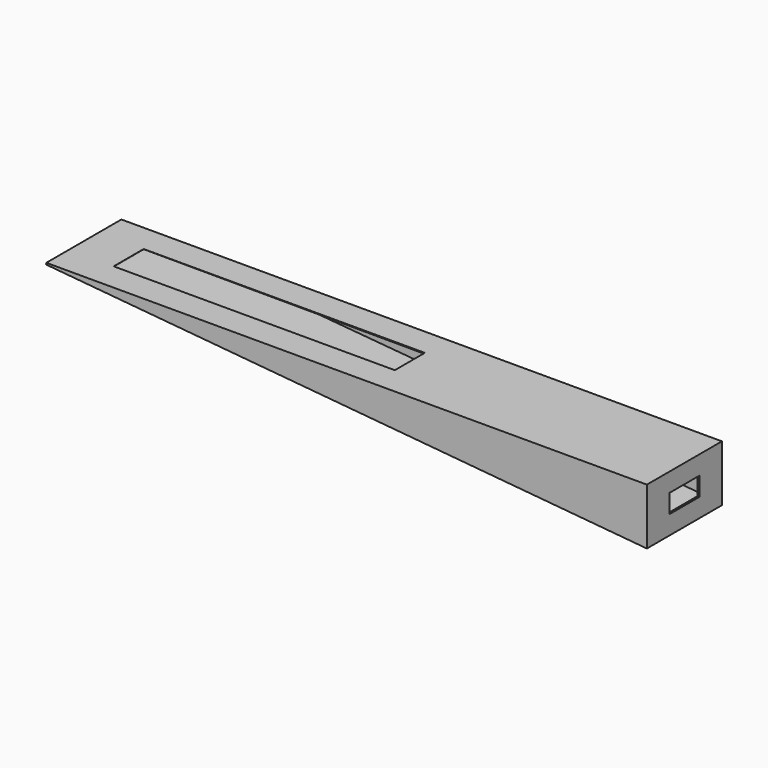
from build123d import *

# Parameters (mm, degrees)
F1_DEPTH = 25
F2_DEPTH = 24.5
F3_W     = 20
F3_H     = 10
F4_DEPTH = 1.061394367
F5_W     = 149.8626496709
F5_H     = 20
F6_DEPTH = 0.5426750459


# Not quite as in the source:
# - a feature names something its author has since deleted; it is built from what else it names


with BuildPart() as f1:
    # F0 (on Front) → F1 (new body, symmetric)
    with BuildSketch(Plane.XZ):
        Polygon((250.3392749669, 0), (-69.6607250331, 0), (-69.7979346905, 0), (-69.9352178344, -0.8798027663), (-69.8012695535, -0.9007038612), (250.3392749669, -30), align=None)
        Polygon((-69.7894617915, -0.8250317769), (-69.6638822556, -0.0320404142), (249.3347435311, -0.9683876885), (249.2535173062, -28.6408707924), align=None, mode=Mode.SUBTRACT)
        Polygon((249.3347435311, -0.9683876885), (-69.6638822556, -0.0320404142), (-69.7894617915, -0.8250317769), (249.2535173062, -28.6408707924), align=None)
    extrude(amount=F1_DEPTH, both=True)

    # F0 (on Front) → F2 (cut, symmetric)
    with BuildSketch(Plane.XZ):
        Polygon((249.3347435311, -0.9683876885), (-69.6638822556, -0.0320404142), (-69.7894617915, -0.8250317769), (249.2535173062, -28.6408707924), align=None)
    extrude(amount=F2_DEPTH, both=True, mode=Mode.SUBTRACT)

    # F3 (on face) → F4 (cut, through all)
    with BuildSketch(Plane.YZ.offset(250.3392749669)):
        with Locations((0, -15)):
            Rectangle(F3_W, F3_H)
    extrude(amount=-F4_DEPTH, mode=Mode.SUBTRACT)

    # F5 (on face) → F6 (cut, through all)
    with BuildSketch(Plane.XY):
        with Locations((29.0292073041, 0)):
            Rectangle(F5_W, F5_H)
    extrude(amount=-F6_DEPTH, mode=Mode.SUBTRACT)


solid = f1.part
